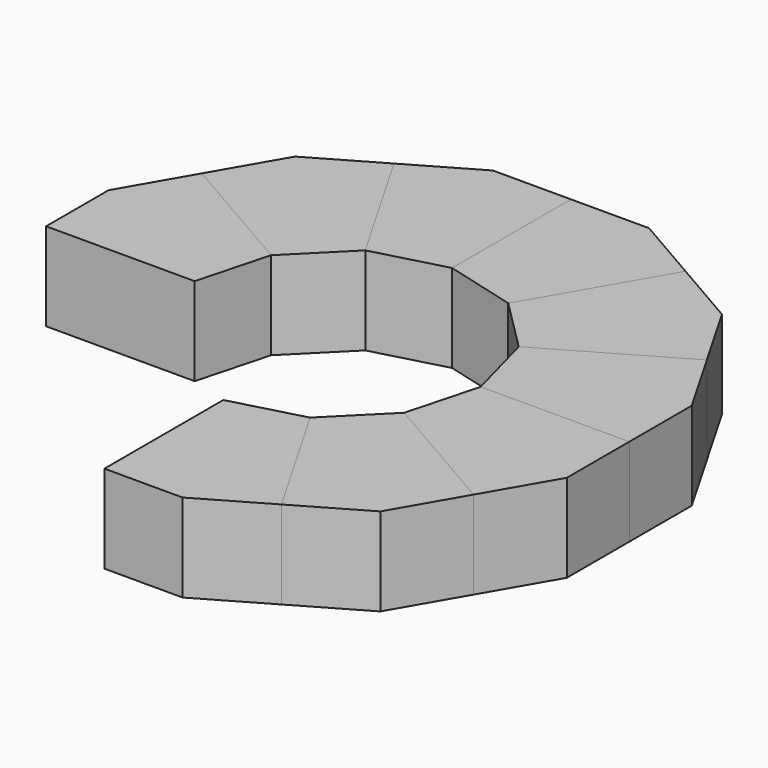
from build123d import *

# Parameters (mm, degrees)
F2_DEPTH = 270.9333333333
F4_COUNT = 9
F4_ANGLE = 240


# Not quite as in the source:
# - a variable given as a bare number and used for a length is read in inches; the dataset says mm whatever the document's units were


with BuildPart() as f2:
    # F0 (on Top) → F2 (new body)
    with BuildSketch(Plane.XY):
        Polygon((-897.1409051225, 0), (-439.9409051225, 0), (-381, 219.9704525612), (-776.9468146102, 448.5704525612), (-897.1409051225, 240.3881810245), align=None)
    extrude(amount=F2_DEPTH)


with BuildPart() as f4_1:
    # F4: instance of F2
    add(f2.part.rotate(Axis((0, 0, 173.5299534571), (0, 0, -1)), 1 * F4_ANGLE / (F4_COUNT - 1)))


with BuildPart() as f4_2:
    # F4: instance of F2
    add(f2.part.rotate(Axis((0, 0, 173.5299534571), (0, 0, -1)), 2 * F4_ANGLE / (F4_COUNT - 1)))


with BuildPart() as f4_3:
    # F4: instance of F2
    add(f2.part.rotate(Axis((0, 0, 173.5299534571), (0, 0, -1)), 3 * F4_ANGLE / (F4_COUNT - 1)))


with BuildPart() as f4_4:
    # F4: instance of F2
    add(f2.part.rotate(Axis((0, 0, 173.5299534571), (0, 0, -1)), 4 * F4_ANGLE / (F4_COUNT - 1)))


with BuildPart() as f4_5:
    # F4: instance of F2
    add(f2.part.rotate(Axis((0, 0, 173.5299534571), (0, 0, -1)), 5 * F4_ANGLE / (F4_COUNT - 1)))


with BuildPart() as f4_6:
    # F4: instance of F2
    add(f2.part.rotate(Axis((0, 0, 173.5299534571), (0, 0, -1)), 6 * F4_ANGLE / (F4_COUNT - 1)))


with BuildPart() as f4_7:
    # F4: instance of F2
    add(f2.part.rotate(Axis((0, 0, 173.5299534571), (0, 0, -1)), 7 * F4_ANGLE / (F4_COUNT - 1)))


with BuildPart() as f4_8:
    # F4: instance of F2
    add(f2.part.rotate(Axis((0, 0, 173.5299534571), (0, 0, -1)), 8 * F4_ANGLE / (F4_COUNT - 1)))


solid = Compound([f2.part, f4_1.part, f4_2.part, f4_3.part, f4_4.part, f4_5.part, f4_6.part, f4_7.part, f4_8.part])
